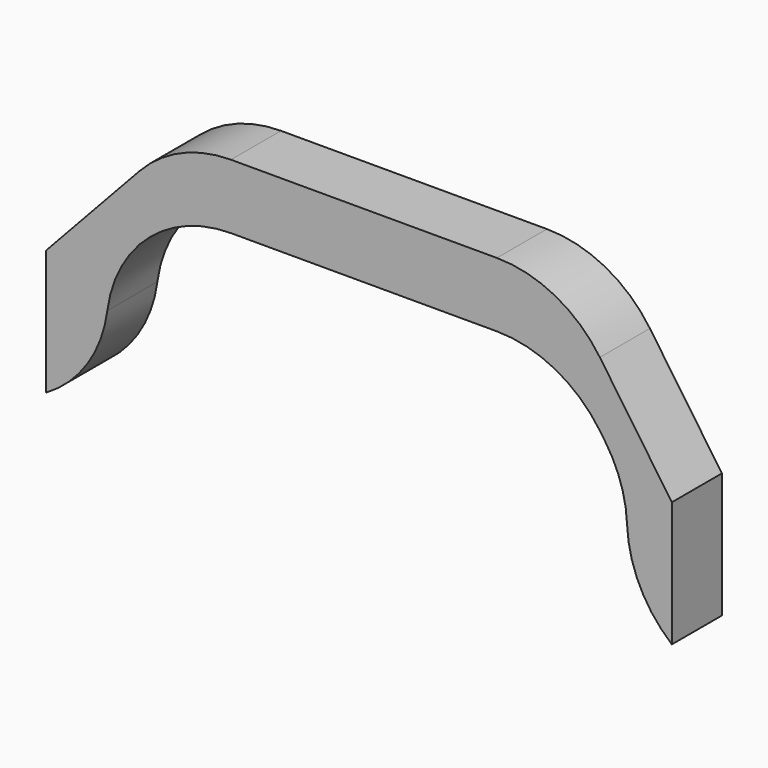
from build123d import *

# Parameters (mm, degrees)
F1_DEPTH    = 2.54
F2_T1_DEPTH = 2.54
F2_T3_DEPTH = 13.5939610314
F2_T5_DEPTH = 15.8607267087
F3_T1_DEPTH = 21.0206169328
F3_T3_DEPTH = 21.2247608177


# Not quite as in the source:
# - a fillet or chamfer that OpenCascade refuses, or shapes differently, is made with other operations: its cross-section is extruded or revolved along the edge and cut away or added


with BuildPart() as f1:
    # F0 (on Front) → F1 (new body)
    with BuildSketch(Plane.XZ):
        Polygon((-31.4589329064, 0), (-36.7512629041, -5.6826620174), (-36.7512629041, -10.7626620174), (-34.308064729, -10.7626620174), (-34.308064729, -5.6826620174), (-31.4589329064, -2.6233945118), (-15.7887097448, -2.6233945118), (-13.1645070408, -6.4200807009), (-13.1645070408, -11.5000807009), (-11.3512629041, -11.5000807009), (-11.3512629041, -6.4200807009), (-15.7887097448, 0), align=None)
    extrude(amount=F1_DEPTH)

    # F2: fillet of radius 5.08 on 6 edges, made by hand

    # F2_s2 → F2_t1 (join)
    with BuildSketch(Plane.XZ):
        with BuildLine():
            ThreePointArc((-32.9656479615, -4.2412362599), (-31.2752859934, -3.0453818498), (-29.2481407001, -2.6233945118))
            Line((-29.2481407001, -2.6233945118), (-31.4589329064, -2.6233945118))
            Line((-31.4589329064, -2.6233945118), (-32.9656479615, -4.2412362599))
        make_face()
        with BuildLine():
            ThreePointArc((-18.4528550865, -2.6233945118), (-16.0934809554, -3.2045331326), (-14.2739191976, -4.8149875397))
            Line((-14.2739191976, -4.8149875397), (-15.7887097448, -2.6233945118))
            Line((-15.7887097448, -2.6233945118), (-18.4528550865, -2.6233945118))
        make_face()
        with BuildLine():
            ThreePointArc((-14.0655711519, -5.1164246759), (-13.3950022045, -6.4919857066), (-13.1645070408, -8.0048316479))
            Line((-13.1645070408, -8.0048316479), (-13.1645070408, -6.4200807009))
            Line((-13.1645070408, -6.4200807009), (-14.0655711519, -5.1164246759))
        make_face()
        with BuildLine():
            ThreePointArc((-34.308064729, -7.6818378518), (-33.9551852525, -5.8215336949), (-32.9455719904, -4.2196795999))
            Line((-32.9455719904, -4.2196795999), (-34.308064729, -5.6826620174))
            Line((-34.308064729, -5.6826620174), (-34.308064729, -7.6818378518))
        make_face()
    extrude(amount=F2_T1_DEPTH)

    # F2_s4 → F2_t3 (cut)
    with BuildSketch(Plane.XZ.offset(-5.5269805157)):
        with BuildLine():
            ThreePointArc((-32.9656479615, -1.6178417481), (-31.2752859934, -0.421987338), (-29.2481407001, 0))
            Line((-29.2481407001, 0), (-31.4589329064, 0))
            Line((-31.4589329064, 0), (-32.9656479615, -1.6178417481))
        make_face()
    extrude(amount=F2_T3_DEPTH, mode=Mode.SUBTRACT)

    # F2_s6 → F2_t5 (cut)
    with BuildSketch(Plane.XZ.offset(-6.6603633543)):
        with BuildLine():
            ThreePointArc((-18.4528550865, 0), (-16.0934809554, -0.5811386208), (-14.2739191976, -2.1915930279))
            Line((-14.2739191976, -2.1915930279), (-15.7887097448, 0))
            Line((-15.7887097448, 0), (-18.4528550865, 0))
        make_face()
    extrude(amount=F2_T5_DEPTH, mode=Mode.SUBTRACT)

    # F3: fillet of radius 5.08 on 2 edges, made by hand

    # F3_s2 → F3_t1 (cut)
    with BuildSketch(Plane.XZ.offset(-9.2403084664)):
        with BuildLine():
            ThreePointArc((-11.3512629041, -11.5000807009), (-12.6512581821, -9.8444473796), (-13.1684800157, -7.8039594497))
            Line((-13.1684800157, -7.8039594497), (-13.6760827182, -7.8240466695))
            ThreePointArc((-13.6760827182, -7.8240466695), (-13.6725070408, -8.0048316479), (-13.6725070408, -11.5000807009))
            Line((-13.6725070408, -11.5000807009), (-13.1645070408, -12.0080807009))
            ThreePointArc((-13.1645070408, -12.0080807009), (-12.2578849724, -12.0080807009), (-11.6771438954, -11.8897800459))
            Line((-11.6771438954, -11.8897800459), (-11.3512629041, -11.5000807009))
        make_face()
    extrude(amount=F3_T1_DEPTH, mode=Mode.SUBTRACT)

    # F3_s4 → F3_t3 (cut)
    with BuildSketch(Plane.XZ.offset(-9.3423804089)):
        with BuildLine():
            ThreePointArc((-34.2655455901, -7.0259517536), (-35.0733800628, -9.183691684), (-36.7512629041, -10.7626620174))
            Line((-36.7512629041, -10.7626620174), (-36.4960865494, -11.2019216536))
            ThreePointArc((-36.4960865494, -11.2019216536), (-35.5296638165, -11.2706620174), (-34.308064729, -11.2706620174))
            Line((-34.308064729, -11.2706620174), (-33.800064729, -10.7626620174))
            ThreePointArc((-33.800064729, -10.7626620174), (-33.800064729, -7.6818378518), (-33.761797504, -7.0915403635))
            Line((-33.761797504, -7.0915403635), (-34.2655455901, -7.0259517536))
        make_face()
    extrude(amount=F3_T3_DEPTH, mode=Mode.SUBTRACT)


solid = f1.part
